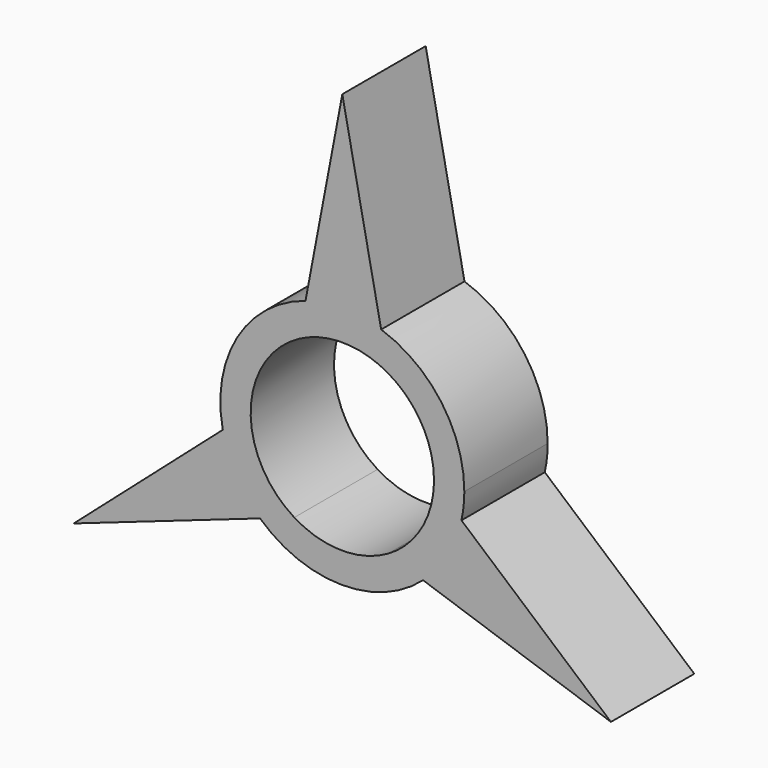
from build123d import *

# Parameters (mm, degrees)
F1_DEPTH = 6.35


with BuildPart() as f1:
    # F0 (on Front) → F1 (new body)
    with BuildSketch(Plane.XZ):
        with BuildLine():
            ThreePointArc((-5.5879735466, 0.0171942529), (-4.7955253497, 2.8685676949), (-2.6580116206, 4.9153553508))
            Line((-2.6580116206, 4.9153553508), (-2.2450949747, 7.0888402589))
            ThreePointArc((-2.2450949747, 7.0888402589), (-6.4075834438, 3.7729275201), (-7.2879952633, -1.4755448838))
            Line((-7.2879952633, -1.4755448838), (-5.5879735466, 0.0171942529))
        make_face()
        with BuildLine():
            ThreePointArc((-2.6580116206, 4.9153553508), (0.0864898214, 5.5873306248), (2.8088774331, 4.8307299206))
            Line((2.8088774331, 4.8307299206), (2.3661382778, 7.0493614826))
            ThreePointArc((2.3661382778, 7.0493614826), (0.0636593572, 7.4355937993), (-2.2450949747, 7.0888402589))
            Line((-2.2450949747, 7.0888402589), (-2.6580116206, 4.9153553508))
        make_face()
        with BuildLine():
            Line((2.3661382778, 7.0493614826), (2.8088774331, 4.8307299206))
            ThreePointArc((2.8088774331, 4.8307299206), (4.8436427973, 2.7865513546), (5.588, 0))
            ThreePointArc((5.588, 0), (5.5874570768, -0.0778936122), (5.5858284127, -0.1557720884))
            Line((5.5858284127, -0.1557720884), (7.2616632349, -1.6001108475))
            ThreePointArc((7.2616632349, -1.6001108475), (7.3921872476, -0.8047828019), (7.435866302, 0))
            ThreePointArc((7.435866302, 0), (6.0368201707, 4.3415331264), (2.3661382778, 7.0493614826))
        make_face()
        with BuildLine():
            ThreePointArc((-2.2450949747, 7.0888402589), (0.0636593572, 7.4355937993), (2.3661382778, 7.0493614826))
            Line((2.3661382778, 7.0493614826), (0, 18.9064312726))
            Line((0, 18.9064312726), (-2.2450949747, 7.0888402589))
        make_face()
        with BuildLine():
            Line((16.373449777, -9.4532156363), (7.2616632349, -1.6001108475))
            ThreePointArc((7.2616632349, -1.6001108475), (6.4075834438, -3.7729275201), (4.9218569854, -5.5738165987))
            Line((4.9218569854, -5.5738165987), (16.373449777, -9.4532156363))
        make_face()
        with BuildLine():
            Line((7.2616632349, -1.6001108475), (5.5858284127, -0.1557720884))
            ThreePointArc((5.5858284127, -0.1557720884), (4.7955253497, -2.8685676949), (2.7790961135, -4.8479241735))
            Line((2.7790961135, -4.8479241735), (4.9218569854, -5.5738165987))
            ThreePointArc((4.9218569854, -5.5738165987), (6.4075834438, -3.7729275201), (7.2616632349, -1.6001108475))
        make_face()
        with BuildLine():
            ThreePointArc((2.7790961135, -4.8479241735), (-0.0864898214, -5.5873306248), (-2.9278167921, -4.7595832624))
            Line((-2.9278167921, -4.7595832624), (-5.0165682602, -5.4887294114))
            ThreePointArc((-5.0165682602, -5.4887294114), (-0.0636593572, -7.4355937993), (4.9218569854, -5.5738165987))
            Line((4.9218569854, -5.5738165987), (2.7790961135, -4.8479241735))
        make_face()
        with BuildLine():
            Line((-16.373449777, -9.4532156363), (-5.0165682602, -5.4887294114))
            ThreePointArc((-5.0165682602, -5.4887294114), (-6.471242801, -3.6626662791), (-7.2879952633, -1.4755448838))
            Line((-7.2879952633, -1.4755448838), (-16.373449777, -9.4532156363))
        make_face()
        with BuildLine():
            Line((-5.0165682602, -5.4887294114), (-2.9278167921, -4.7595832624))
            ThreePointArc((-2.9278167921, -4.7595832624), (-4.8820151711, -2.7187629299), (-5.5879735466, 0.0171942529))
            Line((-5.5879735466, 0.0171942529), (-7.2879952633, -1.4755448838))
            ThreePointArc((-7.2879952633, -1.4755448838), (-6.471242801, -3.6626662791), (-5.0165682602, -5.4887294114))
        make_face()
    extrude(amount=F1_DEPTH)


solid = f1.part
